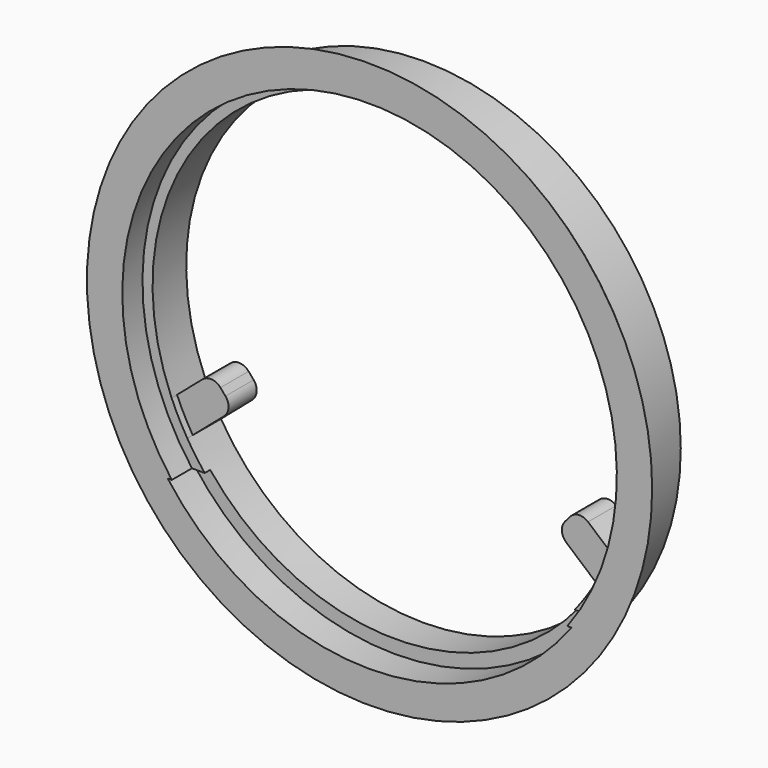
from build123d import *

# Parameters (mm, degrees)
F0_R          = 25.5
F1_DEPTH      = 5.08
F3_R          = 28
F3_R_2        = 23.5
F4_DEPTH      = 1.5875
F5_DEPTH      = 1.5875
F5_DEPTH_BACK = 3.175
F6_DEPTH      = 1.5875
F9_R          = 24.5
F10_DEPTH     = 2.5
F11_R         = 1.27


# Not quite as in the source:
# - a fillet or chamfer that OpenCascade refuses, or shapes differently, is made with other operations: its cross-section is extruded or revolved along the edge and cut away or added


with BuildPart() as f1:
    # F0 (on Front) → F1 (new body)
    with BuildSketch(Plane.XZ):
        Circle(F0_R)
        with BuildLine():
            ThreePointArc((20.0593759089, -12.2421990731), (0, -23.5), (-20.0593759089, -12.2421990731))
            Line((-20.0593759089, -12.2421990731), (-15.990073811, -8.7466746798))
            Line((-15.990073811, -8.7466746798), (-18.1416651056, -6.2419074449))
            Line((-18.1416651056, -6.2419074449), (-21.61384866, -9.2245079057))
            ThreePointArc((-21.61384866, -9.2245079057), (0, 23.5), (21.61384866, -9.2245079057))
            Line((21.61384866, -9.2245079057), (18.1416651056, -6.2419074449))
            Line((18.1416651056, -6.2419074449), (15.990073811, -8.7466746798))
            Line((15.990073811, -8.7466746798), (20.0593759089, -12.2421990731))
        make_face(mode=Mode.SUBTRACT)
    extrude(amount=F1_DEPTH)

    # F3 (on face) → F4 (join)
    with BuildSketch(Plane.XZ.offset(5.08)):
        Circle(F3_R)
        Circle(F3_R_2, mode=Mode.SUBTRACT)
    extrude(amount=F4_DEPTH)

    # F2 (on face) → F5 (cut, two sides)
    with BuildSketch(Plane.XZ.offset(5.08)) as f5_sk:
        with BuildLine():
            Line((20, -14.7076810144), (-20, -14.7076810144))
            ThreePointArc((-20, -14.7076810144), (0, -24.8257100769), (20, -14.7076810144))
        make_face()
    extrude(amount=-F5_DEPTH, mode=Mode.SUBTRACT)
    extrude(f5_sk.sketch, amount=F5_DEPTH_BACK, mode=Mode.SUBTRACT)

    # F6 (cut): faces of the model
    f6_faces = [f1.faces().sort_by_distance(p)[0] for p in [
        (18.9429993018, -5.08, -9.163640961),
        (-18.9429993018, -5.08, -9.163640961),
    ]]
    extrude(f6_faces, amount=-F6_DEPTH, mode=Mode.SUBTRACT)

    # F7: chamfer of 1.5875 on 1 edges, made by hand

    # F7_s1 → F7_t2 (revolve, cut)
    with BuildSketch(Plane.XY):
        Polygon((26.4125, -5.08), (28, -6.6675), (28, -5.08), align=None)
    revolve(axis=Axis((0, -5.08, 0), (0, -1, 0)), mode=Mode.SUBTRACT)

    # F8: fillet of radius 5.08 on 1 edges, made by hand

    # F8_s1 → F8_t2 (revolve, cut)
    with BuildSketch(Plane.XY):
        with BuildLine():
            ThreePointArc((25.5, -5.08), (26.6871185711, -5.586485263), (27.7082857935, -6.3757857935))
            Line((27.7082857935, -6.3757857935), (26.4125, -5.08))
            Line((26.4125, -5.08), (25.5, -5.08))
        make_face()
    revolve(axis=Axis((0, -5.08, 0), (0, -1, 0)), mode=Mode.SUBTRACT)

    # F9 (on face) → F10 (cut)
    with BuildSketch(Plane.XZ.offset(6.6675)):
        Circle(F9_R)
    extrude(amount=-F10_DEPTH, mode=Mode.SUBTRACT)

    # F11
    f11_edges = [f1.edges().sort_by_distance(p)[0] for p in [
        (-15.990074, -1.74625, -8.746675),
        (-18.141665, -1.74625, -6.241907),
        (15.990074, -1.74625, -8.746675),
        (18.141665, -1.74625, -6.241907),
    ]]
    fillet(f11_edges, radius=F11_R)


solid = f1.part
